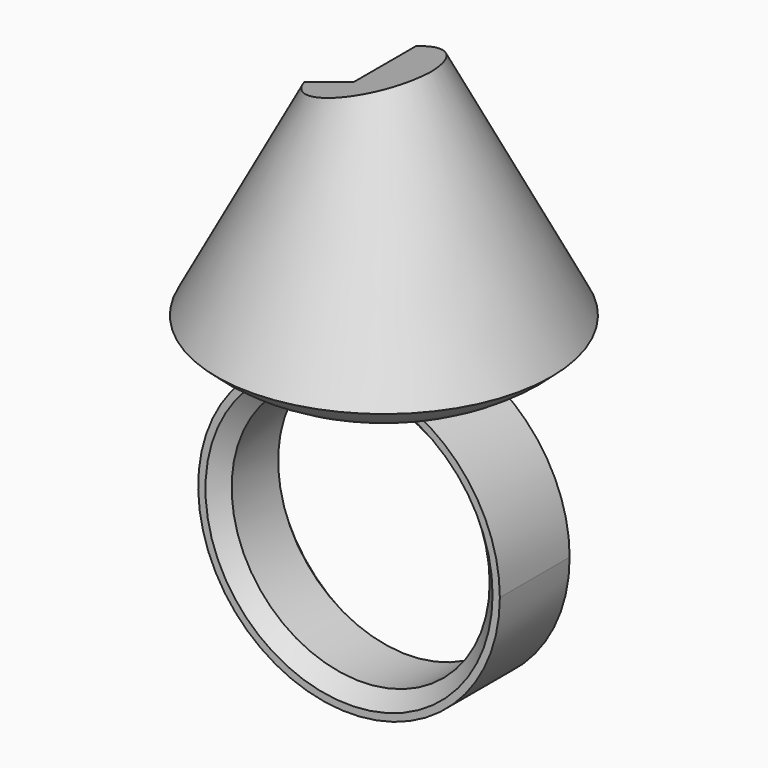
from build123d import *

# Parameters (mm, degrees)
F0_R           = 8.875
F3_DEPTH       = 3
F3_DEPTH_BACK  = 3
F4_SIZE        = 1
F6_DEPTH       = 14.1
F8_START       = 13.5
F7_R           = 4
F7_R_2         = 1.75
F7_R_3         = 0.75
F8_DEPTH       = 6.5
F10_START      = 13
F7_R_4         = 5
F7_R_5         = 4.5
F10_DEPTH      = 8
F11_START      = 13
F11_DEPTH      = 1
F12_START      = 20
F12_DEPTH      = 1
F13_START      = 10.5
F13_DEPTH      = 2.5
F14_START      = 20
F14_DEPTH      = 3.5
F15_START      = 11.5
F15_DEPTH      = 2.5
F16_START      = 20
F16_DEPTH      = 2.5
F20_DEPTH      = 25
F20_DEPTH_BACK = 25


# Not quite as in the source:
# - a feature names something its author has since deleted; it is built from what else it names


with BuildPart() as f2:
    # F0 (on Front) → F2 (revolve)
    with BuildSketch(Plane.XZ):
        with BuildLine():
            ThreePointArc((0, 10.375), (2.3580401671, 10.1034781917), (4.5926568488, 9.3031246401))
            ThreePointArc((4.5926568488, 9.3031246401), (8.3205085843, 10.3091537222), (11.5, 12.5))
            Line((11.5, 12.5), (3.25, 28.3031246401))
            Line((3.25, 28.3031246401), (0, 28.3031246401))
            Line((0, 28.3031246401), (0, 10.375))
        make_face()
    revolve(axis=Axis((0, 0, 0), (0, 0, 1)))

    # F0 (on Front) → F3 (join, two sides)
    with BuildSketch(Plane.XZ) as f3_sk:
        with BuildLine():
            ThreePointArc((0, 10.375), (-7.3362328548, -7.3362328548), (10.375, 0))
            ThreePointArc((10.375, 0), (8.8116241354, 5.4768517505), (4.5926568488, 9.3031246401))
            Line((4.5926568488, 9.3031246401), (0, 9.3031246401))
            Line((0, 9.3031246401), (0, 10.375))
        make_face()
        Circle(F0_R, mode=Mode.SUBTRACT)
        with BuildLine():
            Line((0, 9.3031246401), (4.5926568488, 9.3031246401))
            ThreePointArc((4.5926568488, 9.3031246401), (2.3580401671, 10.1034781917), (0, 10.375))
            Line((0, 10.375), (0, 9.3031246401))
        make_face()
    extrude(amount=F3_DEPTH)
    extrude(f3_sk.sketch, amount=-F3_DEPTH_BACK)

    # F4
    f4_edges = [f2.edges().sort_by_distance(p)[0] for p in [
        (-8.875, -3, 0),
        (-8.875, 3, 0),
    ]]
    chamfer(f4_edges, length=F4_SIZE)

    # F5 (on face) → F6 (cut)
    with BuildSketch(Plane.XY.offset(28.3031246401)):
        with BuildLine():
            Line((-0.8858618094, 14.4863697807), (-16.5064213391, -1.4472623589))
            Line((-16.5064213391, -1.4472623589), (-2.9099710763, -1.4472623589))
            ThreePointArc((-2.9099710763, -1.4472623589), (-2.9720223474, 1.3151361779), (-0.8858618094, 3.1269392151))
            Line((-0.8858618094, 3.1269392151), (-0.8858618094, 14.4863697807))
        make_face()
        with BuildLine():
            ThreePointArc((-0.8858618094, 3.1269392151), (-2.9720223474, 1.3151361779), (-2.9099710763, -1.4472623589))
            Line((-2.9099710763, -1.4472623589), (-0.8858618094, -1.4472623589))
            Line((-0.8858618094, -1.4472623589), (-0.8858618094, 3.1269392151))
        make_face()
    extrude(amount=-F6_DEPTH, mode=Mode.SUBTRACT)

    # F7 (on Top) → F8 (join)
    with BuildSketch(Plane.XY.offset(F8_START)):
        with Locations((1.6641381906, -0.0193633477)):
            Circle(F7_R)
        with Locations((1.6641381906, -0.0193633477)):
            Circle(F7_R_2, mode=Mode.SUBTRACT)
        with Locations((1.6641381906, -0.0193633477)):
            Circle(F7_R_2)
        with Locations((1.6641381906, -0.0193633477)):
            Circle(F7_R_3, mode=Mode.SUBTRACT)
        with Locations((1.6641381906, -0.0193633477)):
            Circle(F7_R_3)
    extrude(amount=F8_DEPTH)

    # F7 (on Top) → F10 (cut)
    with BuildSketch(Plane.XY.offset(F10_START)):
        with Locations((1.6641381906, -0.0193633477)):
            Circle(F7_R_4)
        with Locations((1.6641381906, -0.0193633477)):
            Circle(F7_R_5, mode=Mode.SUBTRACT)
        with Locations((1.6641381906, -0.0193633477)):
            Circle(F7_R_5)
        with Locations((1.6641381906, -0.0193633477)):
            Circle(F7_R, mode=Mode.SUBTRACT)
    extrude(amount=F10_DEPTH, mode=Mode.SUBTRACT)

    # F7 (on Top) → F11 (cut)
    with BuildSketch(Plane.XY.offset(F11_START)):
        with Locations((1.6641381906, -0.0193633477)):
            Circle(F7_R_4)
        with Locations((1.6641381906, -0.0193633477)):
            Circle(F7_R_5, mode=Mode.SUBTRACT)
        with Locations((1.6641381906, -0.0193633477)):
            Circle(F7_R_5)
        with Locations((1.6641381906, -0.0193633477)):
            Circle(F7_R, mode=Mode.SUBTRACT)
        with Locations((1.6641381906, -0.0193633477)):
            Circle(F7_R)
        with Locations((1.6641381906, -0.0193633477)):
            Circle(F7_R_2, mode=Mode.SUBTRACT)
        with Locations((1.6641381906, -0.0193633477)):
            Circle(F7_R_2)
        with Locations((1.6641381906, -0.0193633477)):
            Circle(F7_R_3, mode=Mode.SUBTRACT)
        with Locations((1.6641381906, -0.0193633477)):
            Circle(F7_R_3)
    extrude(amount=F11_DEPTH, mode=Mode.SUBTRACT)

    # F7 (on Top) → F12 (cut)
    with BuildSketch(Plane.XY.offset(F12_START)):
        with Locations((1.6641381906, -0.0193633477)):
            Circle(F7_R_4)
        with Locations((1.6641381906, -0.0193633477)):
            Circle(F7_R_5, mode=Mode.SUBTRACT)
        with Locations((1.6641381906, -0.0193633477)):
            Circle(F7_R_5)
        with Locations((1.6641381906, -0.0193633477)):
            Circle(F7_R, mode=Mode.SUBTRACT)
        with Locations((1.6641381906, -0.0193633477)):
            Circle(F7_R)
        with Locations((1.6641381906, -0.0193633477)):
            Circle(F7_R_2, mode=Mode.SUBTRACT)
        with Locations((1.6641381906, -0.0193633477)):
            Circle(F7_R_2)
        with Locations((1.6641381906, -0.0193633477)):
            Circle(F7_R_3, mode=Mode.SUBTRACT)
        with Locations((1.6641381906, -0.0193633477)):
            Circle(F7_R_3)
    extrude(amount=F12_DEPTH, mode=Mode.SUBTRACT)

    # F7 (on Top) → F13 (cut)
    with BuildSketch(Plane.XY.offset(F13_START)):
        with Locations((1.6641381906, -0.0193633477)):
            Circle(F7_R_2)
        with Locations((1.6641381906, -0.0193633477)):
            Circle(F7_R_3, mode=Mode.SUBTRACT)
        with Locations((1.6641381906, -0.0193633477)):
            Circle(F7_R_3)
    extrude(amount=F13_DEPTH, mode=Mode.SUBTRACT)

    # F7 (on Top) → F14 (cut)
    with BuildSketch(Plane.XY.offset(F14_START)):
        with Locations((1.6641381906, -0.0193633477)):
            Circle(F7_R_2)
        with Locations((1.6641381906, -0.0193633477)):
            Circle(F7_R_3, mode=Mode.SUBTRACT)
        with Locations((1.6641381906, -0.0193633477)):
            Circle(F7_R_3)
    extrude(amount=F14_DEPTH, mode=Mode.SUBTRACT)

    # F7 (on Top) → F15 (join)
    with BuildSketch(Plane.XY.offset(F15_START)):
        with Locations((1.6641381906, -0.0193633477)):
            Circle(F7_R_3)
    extrude(amount=F15_DEPTH)

    # F7 (on Top) → F16 (join)
    with BuildSketch(Plane.XY.offset(F16_START)):
        with Locations((1.6641381906, -0.0193633477)):
            Circle(F7_R_3)
    extrude(amount=F16_DEPTH)

    # F19 (on Front) → F20 (cut, two sides)
    with BuildSketch(Plane.XZ) as f20_sk:
        Polygon((-4.3850070654, 28.8974568248), (-4.594437778, 25.7020443678), (4.991795402, 28.8974568248), align=None)
    extrude(amount=-F20_DEPTH, mode=Mode.SUBTRACT)
    extrude(f20_sk.sketch, amount=F20_DEPTH_BACK, mode=Mode.SUBTRACT)


solid = f2.part
